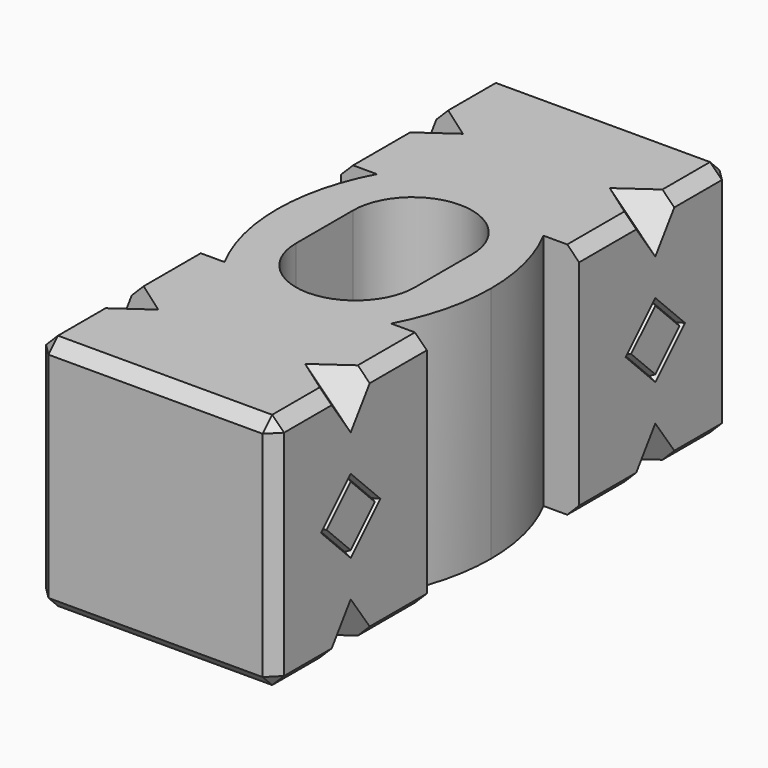
from build123d import *

# Parameters (mm, degrees)
F0_W              = 31.75
F0_H              = 31.75
F1_DEPTH          = 38.1
F2_SIZE           = 1.5875
F4_DEPTH          = 31.751
F7_DEPTH          = 12.7
F10_DEPTH         = 12.7
F13_COPIES2_COUNT = 2


# Not quite as in the source:
# - a pattern or mirror of a feature is missing from the dataset's text; its kind, count and spacing are read off the source's solid


with BuildPart() as f1:
    # F0 (on Front) → F1 (new body, symmetric)
    with BuildSketch(Plane.XZ):
        Rectangle(F0_W, F0_H)
    extrude(amount=F1_DEPTH, both=True)

    # F2
    f2_edges = [f1.edges().sort_by_distance(p)[0] for p in [
        (0, -38.1, 15.875),
        (15.875, -38.1, 0),
        (15.875, 0, 15.875),
        (15.875, 0, -15.875),
        (-15.875, 0, 15.875),
        (-15.875, -38.1, 0),
        (0, -38.1, -15.875),
        (15.875, 38.1, 0),
        (-15.875, 38.1, 0),
        (0, 38.1, -15.875),
        (-15.875, 0, -15.875),
        (0, 38.1, 15.875),
    ]]
    chamfer(f2_edges, length=F2_SIZE)

    # F3 (on face) → F4 (cut, through all)
    with BuildSketch(Plane.XY.offset(15.875)):
        with BuildLine():
            Line((11.1125, -12.7), (14.2875, -12.7))
            Line((14.2875, -12.7), (14.2875, 1.197e-07))
            ThreePointArc((14.2875, 1.197e-07), (13.4817207372, -6.5454301226), (11.1125, -12.7))
        make_face()
        Polygon((14.2875, 1.197e-07), (14.2875, -12.7), (15.875, -12.7), (15.875, 12.7), (14.2875, 12.7), align=None)
        with BuildLine():
            ThreePointArc((11.1125, 12.7), (13.4817207082, 6.5454302387), (14.2875, 1.197e-07))
            Line((14.2875, 1.197e-07), (14.2875, 12.7))
            Line((14.2875, 12.7), (11.1125, 12.7))
        make_face()
        Polygon((-15.875, -12.7), (-14.2875, -12.7), (-14.2875, 1.197e-07), (-14.2875, 12.7), (-15.875, 12.7), align=None)
        with BuildLine():
            Line((-14.2875, 1.197e-07), (-14.2875, -12.7))
            Line((-14.2875, -12.7), (-11.1125, -12.7))
            ThreePointArc((-11.1125, -12.7), (-13.4817207372, -6.5454301226), (-14.2875, 1.197e-07))
        make_face()
        with BuildLine():
            Line((-14.2875, 12.7), (-14.2875, 1.197e-07))
            ThreePointArc((-14.2875, 1.197e-07), (-13.4817207082, 6.5454302387), (-11.1125, 12.7))
            Line((-11.1125, 12.7), (-14.2875, 12.7))
        make_face()
        with BuildLine():
            Line((-7.9375, 4.7625), (-7.9375, -4.7625))
            ThreePointArc((-7.9375, -4.7625), (0, -12.7), (7.9375, -4.7625))
            Line((7.9375, -4.7625), (7.9375, 4.7625))
            ThreePointArc((7.9375, 4.7625), (0, 12.7), (-7.9375, 4.7625))
        make_face()
    extrude(amount=-F4_DEPTH, mode=Mode.SUBTRACT)

    # F6 (on face) → F7 (cut, symmetric)
    with BuildSketch(Plane(origin=(0, 0, 0), x_dir=(0, 1, 0), z_dir=(0.7071067812, 0, 0.7071067812))):
        Polygon((-25.4, 18.1531082875), (-22.225, 21.3281082875), (-28.575, 21.3281082875), align=None)
        Polygon((-25.4, -18.1531082875), (-28.575, -21.3281082875), (-22.225, -21.3281082875), align=None)
        Polygon((22.225, -21.3281082875), (28.575, -21.3281082875), (25.4, -18.1531082875), align=None)
        Polygon((28.575, 21.3281082875), (22.225, 21.3281082875), (25.4, 18.1531082875), align=None)
    extrude(amount=F7_DEPTH, both=True, mode=Mode.SUBTRACT)

    # F9 (on face) → F10 (cut, symmetric)
    with BuildSketch(Plane(origin=(0, 0, 0), x_dir=(0, 1, 0), z_dir=(0.7071067812, 0, -0.7071067812))):
        Polygon((-25.4, 18.1531082875), (-22.225, 21.3281082875), (-28.575, 21.3281082875), align=None)
        Polygon((-28.575, -21.3281082875), (-22.225, -21.3281082875), (-25.4, -18.1531082875), align=None)
        Polygon((28.575, 21.3281082875), (22.225, 21.3281082875), (25.4, 18.1531082875), align=None)
        Polygon((25.4, -18.1531082875), (22.225, -21.3281082875), (28.575, -21.3281082875), align=None)
    extrude(amount=F10_DEPTH, both=True, mode=Mode.SUBTRACT)

    # F13: sweep along a path in F11
    with BuildLine(Plane(origin=(-15.875, 0, 0), x_dir=(0, -1, 0), z_dir=(-1, 0, 0))) as f13_path:
        Line((-25.4, 4.4901280605), (-29.8901280605, 0))
        Line((-29.8901280605, 0), (-25.4, -4.4901280605))
        Line((-25.4, -4.4901280605), (-20.9098719395, 0))
        Line((-20.9098719395, 0), (-25.4, 4.4901280605))
    # F12 (on Top) → F13 (sweep, cut)
    with BuildSketch(Plane.XY):
        Polygon((-15.875, 29.4318562844), (-15.08125, 29.8901280605), (-15.875, 30.3483998367), align=None)
    f13 = sweep(path=f13_path.line, transition=Transition.RIGHT, mode=Mode.SUBTRACT)

    # F13_copies: F13 across plane
    add(f13.mirror(Plane(origin=(0, 0, 0), x_dir=(0, 0, 1), z_dir=(1, 0, 0))), mode=Mode.SUBTRACT)

    # F13_copies1: F13 across plane
    add(f13.mirror(Plane(origin=(0, 0, 0), x_dir=(0, 0, -1), z_dir=(0, -1, 0))), mode=Mode.SUBTRACT)

    # F13_copies2: F13 ×2 about axis
    f13_copies2_axis = Axis((0, 0, 0), (0, 0, 1))
    for i in range(1, F13_COPIES2_COUNT):
        add(f13.rotate(f13_copies2_axis, i * 360 / F13_COPIES2_COUNT), mode=Mode.SUBTRACT)


solid = f1.part
